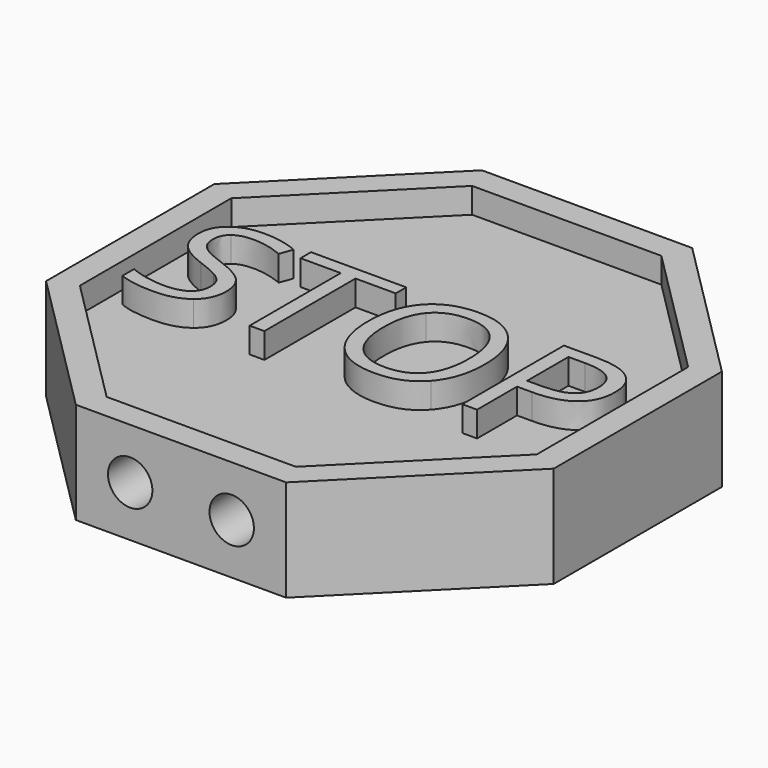
from build123d import *

# Parameters (mm, degrees)
F1_DEPTH = 8
F3_DEPTH = 2
F5_D     = 3.5
F5_DEPTH = 8
F5_TIP   = 1.0515060833


with BuildPart() as f1:
    # F0 (on Top) → F1 (new body)
    with BuildSketch(Plane.XY):
        Polygon((20, -8.2842712475), (20, 8.2842712475), (8.2842712475, 20), (-8.2842712475, 20), (-20, 8.2842712475), (-20, -8.2842712475), (-8.2842712475, -20), (8.2842712475, -20), align=None)
    extrude(amount=F1_DEPTH)

    # F2 (on face) → F3 (cut)
    with BuildSketch(Plane.XY.offset(8)):
        Polygon((18, -7.4558441227), (18, 7.4558441227), (7.4558441227, 18), (-7.4558441227, 18), (-18, 7.4558441227), (-18, -7.4558441227), (-7.4558441227, -18), (7.4558441227, -18), align=None)
        with BuildLine():
            add(Edge.make_bspline(
                [(-11.0686569032, -0.7610464389), (-10.4772186757, -1.4050569533), (-10.4772186757, -2.4302165478)],
                knots=[0, 0, 0, 1, 1, 1], degree=2))
            add(Edge.make_bspline(
                [(-10.4772186757, -2.4302165478), (-10.4772186757, -3.751095256), (-11.4355676555, -4.4914882964)],
                knots=[0, 0, 0, 1, 1, 1], degree=2))
            add(Edge.make_bspline(
                [(-11.4355676555, -4.4914882964), (-12.3939166354, -5.2318813368), (-14.0368006008, -5.2318813368)],
                knots=[0, 0, 0, 1, 1, 1], degree=2))
            add(Edge.make_bspline(
                [(-14.0368006008, -5.2318813368), (-15.8154963074, -5.2318813368), (-16.7749405432, -4.7718738265)],
                knots=[0, 0, 0, 1, 1, 1], degree=2))
            Line((-16.7749405432, -4.7718738265), (-16.7749405432, -3.6503317061))
            add(Edge.make_bspline(
                [(-16.7749405432, -3.6503317061), (-16.1572161722, -3.9088121167), (-15.4321567155, -4.0599574415)],
                knots=[0, 0, 0, 1, 1, 1], degree=2))
            add(Edge.make_bspline(
                [(-15.4321567155, -4.0599574415), (-14.7070972587, -4.2111027663), (-13.9951808737, -4.2111027663)],
                knots=[0, 0, 0, 1, 1, 1], degree=2))
            add(Edge.make_bspline(
                [(-13.9951808737, -4.2111027663), (-12.8320190262, -4.2111027663), (-12.2427713106, -3.7697146076)],
                knots=[0, 0, 0, 1, 1, 1], degree=2))
            add(Edge.make_bspline(
                [(-12.2427713106, -3.7697146076), (-11.6535235949, -3.3283264489), (-11.6535235949, -2.5397421454)],
                knots=[0, 0, 0, 1, 1, 1], degree=2))
            add(Edge.make_bspline(
                [(-11.6535235949, -2.5397421454), (-11.6535235949, -2.0205908124), (-11.8627174865, -1.6887282513)],
                knots=[0, 0, 0, 1, 1, 1], degree=2))
            add(Edge.make_bspline(
                [(-11.8627174865, -1.6887282513), (-12.0719113781, -1.3568656903), (-12.5614907998, -1.0753849042)],
                knots=[0, 0, 0, 1, 1, 1], degree=2))
            add(Edge.make_bspline(
                [(-12.5614907998, -1.0753849042), (-13.0510702216, -0.7939041182), (-14.0499436725, -0.4390411816)],
                knots=[0, 0, 0, 1, 1, 1], degree=2))
            add(Edge.make_bspline(
                [(-14.0499436725, -0.4390411816), (-15.4452997872, 0.0603955439), (-16.0444048066, 0.7449305295)],
                knots=[0, 0, 0, 1, 1, 1], degree=2))
            add(Edge.make_bspline(
                [(-16.0444048066, 0.7449305295), (-16.643509826, 1.4294655151), (-16.643509826, 2.5312930279)],
                knots=[0, 0, 0, 1, 1, 1], degree=2))
            add(Edge.make_bspline(
                [(-16.643509826, 2.5312930279), (-16.643509826, 3.6878833396), (-15.7749718363, 4.3724183252)],
                knots=[0, 0, 0, 1, 1, 1], degree=2))
            add(Edge.make_bspline(
                [(-15.7749718363, 4.3724183252), (-14.9064338465, 5.0569533108), (-13.4738390287, 5.0569533108)],
                knots=[0, 0, 0, 1, 1, 1], degree=2))
            add(Edge.make_bspline(
                [(-13.4738390287, 5.0569533108), (-11.982100388, 5.0569533108), (-10.7291275504, 4.5093253223)],
                knots=[0, 0, 0, 1, 1, 1], degree=2))
            Line((-10.7291275504, 4.5093253223), (-11.0927525347, 3.4973087996))
            add(Edge.make_bspline(
                [(-11.0927525347, 3.4973087996), (-12.3325823007, 4.0164601327), (-13.5023156841, 4.0164601327)],
                knots=[0, 0, 0, 1, 1, 1], degree=2))
            add(Edge.make_bspline(
                [(-13.5023156841, 4.0164601327), (-14.4267117286, 4.0164601327), (-14.9469583177, 3.619977469)],
                knots=[0, 0, 0, 1, 1, 1], degree=2))
            add(Edge.make_bspline(
                [(-14.9469583177, 3.619977469), (-15.4672049067, 3.2234948054), (-15.4672049067, 2.5181499562)],
                knots=[0, 0, 0, 1, 1, 1], degree=2))
            add(Edge.make_bspline(
                [(-15.4672049067, 2.5181499562), (-15.4672049067, 1.9989986231), (-15.2755351108, 1.6660408061)],
                knots=[0, 0, 0, 1, 1, 1], degree=2))
            add(Edge.make_bspline(
                [(-15.2755351108, 1.6660408061), (-15.0838653148, 1.3330829891), (-14.6282388284, 1.0559832269)],
                knots=[0, 0, 0, 1, 1, 1], degree=2))
            add(Edge.make_bspline(
                [(-14.6282388284, 1.0559832269), (-14.172612342, 0.7788834648), (-13.2350732257, 0.4437351358)],
                knots=[0, 0, 0, 1, 1, 1], degree=2))
            add(Edge.make_bspline(
                [(-13.2350732257, 0.4437351358), (-11.6600951308, -0.1170359244), (-11.0686569032, -0.7610464389)],
                knots=[0, 0, 0, 1, 1, 1], degree=2))
        make_face(mode=Mode.SUBTRACT)
        Polygon((-5.3492301915, 3.8806483915), (-5.3492301915, -5.0938790837), (-6.5123920391, -5.0938790837), (-6.5123920391, 3.8806483915), (-9.6820628364, 3.8806483915), (-9.6820628364, 4.9145700338), (-2.1795593942, 4.9145700338), (-2.1795593942, 3.8806483915), align=None, mode=Mode.SUBTRACT)
        with BuildLine():
            add(Edge.make_bspline(
                [(6.8037301289, 3.7032169233), (8.0150832395, 2.3341469521), (8.0150832395, -0.0754161973)],
                knots=[0, 0, 0, 1, 1, 1], degree=2))
            add(Edge.make_bspline(
                [(8.0150832395, -0.0754161973), (8.0150832395, -2.4784078107), (6.799349105, -3.8551445738)],
                knots=[0, 0, 0, 1, 1, 1], degree=2))
            add(Edge.make_bspline(
                [(6.799349105, -3.8551445738), (5.5836149706, -5.2318813368), (3.421579672, -5.2318813368)],
                knots=[0, 0, 0, 1, 1, 1], degree=2))
            add(Edge.make_bspline(
                [(3.421579672, -5.2318813368), (1.2113531105, -5.2318813368), (0.0098573038, -3.8792402053)],
                knots=[0, 0, 0, 1, 1, 1], degree=2))
            add(Edge.make_bspline(
                [(0.0098573038, -3.8792402053), (-1.1916385029, -2.5265990737), (-1.1916385029, -0.0622731255)],
                knots=[0, 0, 0, 1, 1, 1], degree=2))
            add(Edge.make_bspline(
                [(-1.1916385029, -0.0622731255), (-1.1916385029, 2.382338215), (0.0131430717, 3.7273125548)],
                knots=[0, 0, 0, 1, 1, 1], degree=2))
            add(Edge.make_bspline(
                [(0.0131430717, 3.7273125548), (1.2179246464, 5.0722868945), (3.4347227438, 5.0722868945)],
                knots=[0, 0, 0, 1, 1, 1], degree=2))
            add(Edge.make_bspline(
                [(3.4347227438, 5.0722868945), (5.5923770184, 5.0722868945), (6.8037301289, 3.7032169233)],
                knots=[0, 0, 0, 1, 1, 1], degree=2))
        make_face(mode=Mode.SUBTRACT)
        with BuildLine():
            add(Edge.make_bspline(
                [(12.840781074, 4.9145700338), (16.5909375391, 4.9145700338), (16.5909375391, 1.9989986231)],
                knots=[0, 0, 0, 1, 1, 1], degree=2))
            add(Edge.make_bspline(
                [(16.5909375391, 1.9989986231), (16.5909375391, 0.4787833271), (15.5537301289, -0.3393728877)],
                knots=[0, 0, 0, 1, 1, 1], degree=2))
            add(Edge.make_bspline(
                [(15.5537301289, -0.3393728877), (14.5165227187, -1.1575291025), (12.5866816873, -1.1575291025)],
                knots=[0, 0, 0, 1, 1, 1], degree=2))
            Line((12.5866816873, -1.1575291025), (11.4081862561, -1.1575291025))
            Line((11.4081862561, -1.1575291025), (11.4081862561, -5.0938790837))
            Line((11.4081862561, -5.0938790837), (10.2450244086, -5.0938790837))
            Line((10.2450244086, -5.0938790837), (10.2450244086, 4.9145700338))
            Line((10.2450244086, 4.9145700338), (12.840781074, 4.9145700338))
        make_face(mode=Mode.SUBTRACT)
        with BuildLine():
            add(Edge.make_bspline(
                [(0.905776693, 2.9803479785), (0.0394292152, 1.9289022406), (0.0394292152, -0.0754161973)],
                knots=[0, 0, 0, 1, 1, 1], degree=2))
            add(Edge.make_bspline(
                [(0.0394292152, -0.0754161973), (0.0394292152, -2.1082112905), (0.905776693, -3.1596570284)],
                knots=[0, 0, 0, 1, 1, 1], degree=2))
            add(Edge.make_bspline(
                [(0.905776693, -3.1596570284), (1.7721241707, -4.2111027663), (3.421579672, -4.2111027663)],
                knots=[0, 0, 0, 1, 1, 1], degree=2))
            add(Edge.make_bspline(
                [(3.421579672, -4.2111027663), (5.0841782451, -4.2111027663), (5.9330016272, -3.1640380523)],
                knots=[0, 0, 0, 1, 1, 1], degree=2))
            add(Edge.make_bspline(
                [(5.9330016272, -3.1640380523), (6.7818250094, -2.1169733383), (6.7818250094, -0.0754161973)],
                knots=[0, 0, 0, 1, 1, 1], degree=2))
            add(Edge.make_bspline(
                [(6.7818250094, -0.0754161973), (6.7818250094, 1.9442358243), (5.9362873952, 2.9880147703)],
                knots=[0, 0, 0, 1, 1, 1], degree=2))
            add(Edge.make_bspline(
                [(5.9362873952, 2.9880147703), (5.0907497809, 4.0317937164), (3.4347227438, 4.0317937164)],
                knots=[0, 0, 0, 1, 1, 1], degree=2))
            add(Edge.make_bspline(
                [(3.4347227438, 4.0317937164), (1.7721241707, 4.0317937164), (0.905776693, 2.9803479785)],
                knots=[0, 0, 0, 1, 1, 1], degree=2))
        make_face()
        with BuildLine():
            Line((11.4081862561, 3.906934535), (11.4081862561, -0.1586556515))
            Line((11.4081862561, -0.1586556515), (12.457441482, -0.1586556515))
            add(Edge.make_bspline(
                [(12.457441482, -0.1586556515), (14.0039429215, -0.1586556515), (14.695049443, 0.340781074)],
                knots=[0, 0, 0, 1, 1, 1], degree=2))
            add(Edge.make_bspline(
                [(14.695049443, 0.340781074), (15.3861559645, 0.8402177995), (15.3861559645, 1.9442358243)],
                knots=[0, 0, 0, 1, 1, 1], degree=2))
            add(Edge.make_bspline(
                [(15.3861559645, 1.9442358243), (15.3861559645, 2.9365377394), (14.7355739141, 3.4217361372)],
                knots=[0, 0, 0, 1, 1, 1], degree=2))
            add(Edge.make_bspline(
                [(14.7355739141, 3.4217361372), (14.0849918638, 3.906934535), (12.7093503567, 3.906934535)],
                knots=[0, 0, 0, 1, 1, 1], degree=2))
            Line((12.7093503567, 3.906934535), (11.4081862561, 3.906934535))
        make_face()
    extrude(amount=-F3_DEPTH, mode=Mode.SUBTRACT)

    # F5
    with Locations(Plane.XZ.offset(20)):
        with Locations((-4, 4), (4, 4)):
            Hole(F5_D / 2, depth=F5_DEPTH)
            with Locations((0, 0, -(F5_DEPTH + F5_TIP / 2))):  # 118° drill point
                Cone(0, F5_D / 2, F5_TIP, mode=Mode.SUBTRACT)


solid = f1.part
